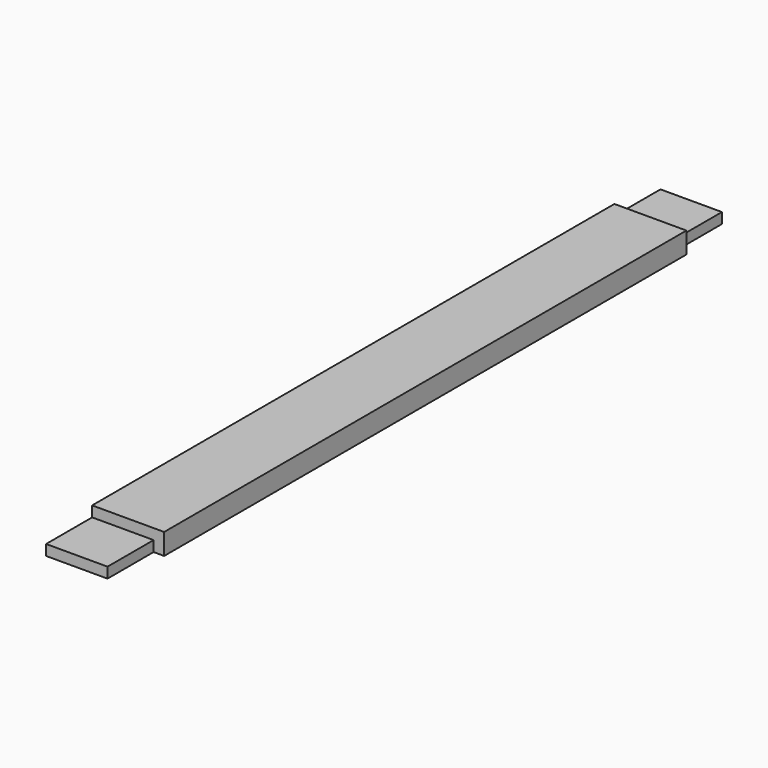
from build123d import *

# Parameters (mm, degrees)
F0_W     = 150
F0_H     = 44
F1_DEPTH = 1600
F4_W     = 22
F4_H     = 120
F5_DEPTH = 44
F6_W     = 128
F6_H     = 120
F7_DEPTH = 22


# Not quite as in the source:
# - a pattern or mirror of a feature is missing from the dataset's text; its kind, count and spacing are read off the source's solid


with BuildPart() as f1:
    # F0 (on Front) → F1 (new body)
    with BuildSketch(Plane.XZ):
        with Locations((-75, 22)):
            Rectangle(F0_W, F0_H)
    extrude(amount=-F1_DEPTH)

    # F4 (on face) → F5 (cut, through all)
    with BuildSketch(Plane.XY.offset(44)):
        with Locations((-11, 1540)):
            Rectangle(F4_W, F4_H)
    f5 = extrude(amount=-F5_DEPTH, mode=Mode.SUBTRACT)

    # F5_copies: F5 across plane
    add(f5.mirror(Plane(origin=(0, 800, 0), x_dir=(0, 0, -1), z_dir=(0, -1, 0))), mode=Mode.SUBTRACT)

    # F6 (on face) → F7 (cut)
    with BuildSketch(Plane.XY.offset(44)):
        with Locations((-86, 1540)):
            Rectangle(F6_W, F6_H)
    f7 = extrude(amount=-F7_DEPTH, mode=Mode.SUBTRACT)

    # F7_copies: F7 across plane
    add(f7.mirror(Plane(origin=(0, 800, 0), x_dir=(0, 0, -1), z_dir=(0, -1, 0))), mode=Mode.SUBTRACT)


solid = f1.part
